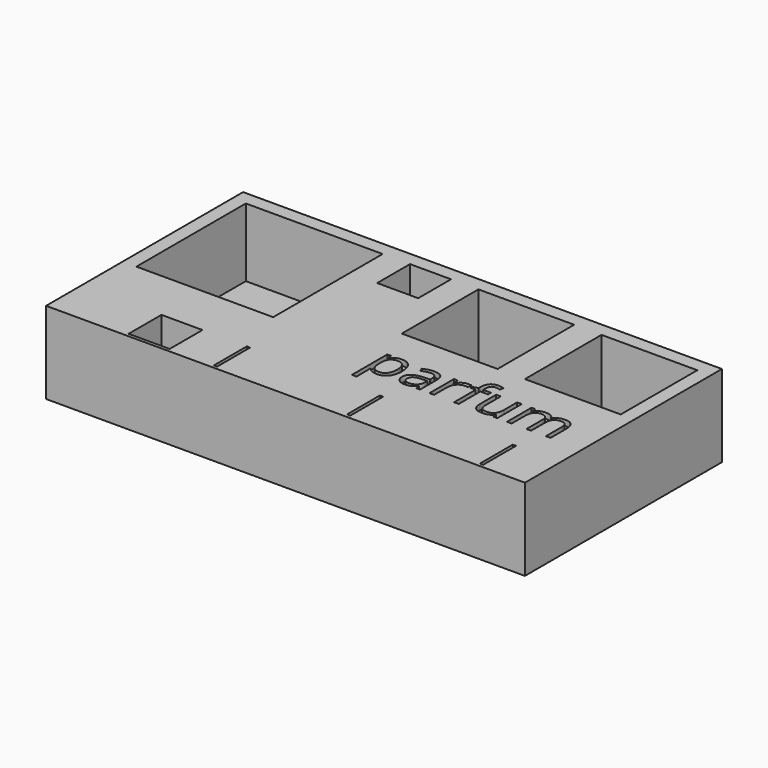
from build123d import *

# Parameters (mm, degrees)
F0_W         = 175
F0_H         = 90
F1_DEPTH     = 30
F2_W         = 1.2
F2_H         = 15
F2_W_2       = 35
F2_H_2       = 35
F2_W_3       = 15
F2_W_4       = 6.8
F2_H_3       = 50
F2_W_5       = 43.2
F3_DEPTH     = 25
F5_TEXT_SIZE = 20.8333333333
F6_DEPTH     = 2


# Not quite as in the source:
# - a feature names something its author has since deleted; it is built from what else it names
# - Text() gives the source's letters only with a copy of the font that has no kerning and outlines rounded to 1/6400 em; it was checked with that copy


with BuildPart() as f1:
    # F0 (on Top) → F1 (new body)
    with BuildSketch(Plane.XY):
        with Locations((-87.5, -45)):
            Rectangle(F0_W, F0_H)
    extrude(amount=F1_DEPTH)

    # F2 (on face) → F3 (cut)
    with BuildSketch(Plane.XY.offset(30)):
        Polygon((-130.8, -73.8), (-145.8, -73.8), (-145.8, -88.8), (-140, -88.8), (-130.8, -88.8), align=None)
        with Locations((-114, -81.3)):
            Rectangle(F2_W, F2_H)
        with Locations((-65.4, -81.3)):
            Rectangle(F2_W, F2_H)
        with Locations((-16.8, -81.3)):
            Rectangle(F2_W, F2_H)
        with Locations((-22.5, -22.5)):
            Rectangle(F2_W_2, F2_H_2)
        with Locations((-67.5, -22.5)):
            Rectangle(F2_W_2, F2_H_2)
        with Locations((-102.5, -12.5)):
            Rectangle(F2_W_3, F2_H)
        with Locations((-166.6, -30)):
            Rectangle(F2_W_4, F2_H_3)
        with Locations((-141.6, -30)):
            Rectangle(F2_W_5, F2_H_3)
    extrude(amount=-F3_DEPTH, mode=Mode.SUBTRACT)

    # F5 (on face) → F6 (cut)
    with BuildSketch(Plane.XY.offset(30)):
        with Locations((-81.9777520088, -63.8)):
            Text('parfum', F5_TEXT_SIZE, font='Open Sans', text_align=(TextAlign.LEFT, TextAlign.BOTTOM))
    extrude(amount=-F6_DEPTH, mode=Mode.SUBTRACT)


solid = f1.part
